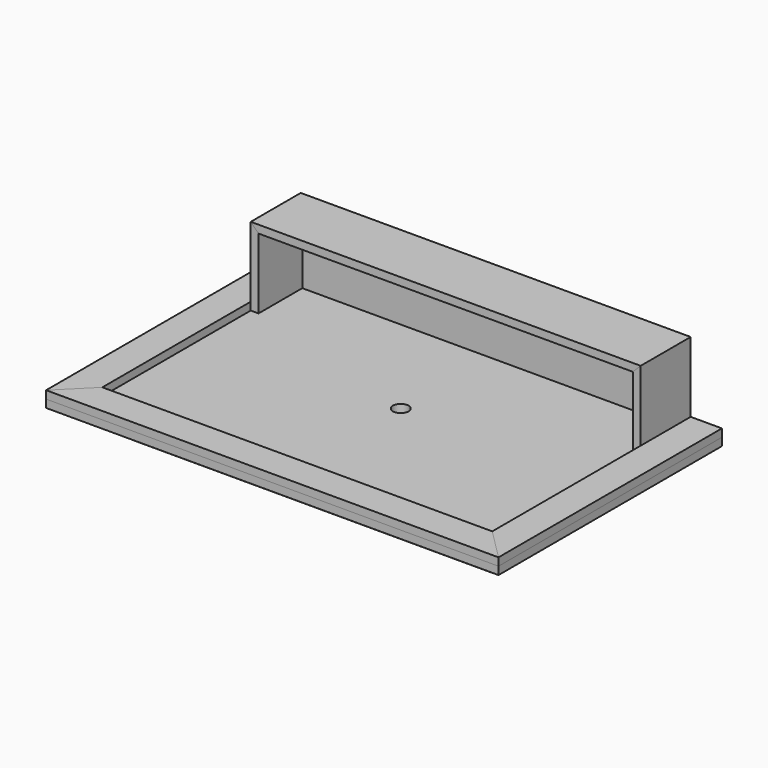
from build123d import *

# Parameters (mm, degrees)
F0_W      = 1470.6092
F0_H      = 907.74012
F1_DEPTH  = 25.4
F2_W      = 1165.8091658585
F2_H      = 720.8011658585
F2_W_2    = 1115.0092
F2_H_2    = 670.0012
F3_DEPTH  = 107.95
F4_R      = 25.4
F5_DEPTH  = 25.4
F6_R      = 9.525
F7_DEPTH  = 720.8011658585
F9_DEPTH  = 25.4
F10_DEPTH = 25.4
F11_DEPTH = 25.4
F12_W     = 1216.6092
F12_H     = 25.4
F13_DEPTH = 254
F14_SIZE  = 25.39999
F16_W     = 1267.4092
F16_H     = 203.2
F17_DEPTH = 25.4
F18_SIZE  = 25.39999


# Not quite as in the source:
# - a fillet or chamfer is up to 0.001 mm smaller than in the source, because OpenCascade refuses the exact size


with BuildPart() as f1:
    # F0 (on Top) → F1 (new body)
    with BuildSketch(Plane.XY):
        with Locations((735.3046, -453.87006)):
            Rectangle(F0_W, F0_H)
    extrude(amount=F1_DEPTH)

    # F2 (on face) → F3 (join)
    with BuildSketch(Plane(origin=(0, 0, 0), x_dir=(1, 0, 0), z_dir=(0, 0, -1))):
        with Locations((735.3046, 385.8005829292)):
            Rectangle(F2_W, F2_H)
        with Locations((735.3046, 385.8005829292)):
            Rectangle(F2_W_2, F2_H_2, mode=Mode.SUBTRACT)
    extrude(amount=F3_DEPTH)

    # F4 (on face) → F5 (cut, through all)
    with BuildSketch(Plane(origin=(0, 0, 0), x_dir=(1, 0, 0), z_dir=(0, 0, -1))):
        with Locations((735.3046, 385.8005829292)):
            Circle(F4_R)
    extrude(amount=-F5_DEPTH, mode=Mode.SUBTRACT)

    # F6 (on face) → F7 (cut, through all)
    with BuildSketch(Plane.XZ.offset(746.2011658585)):
        with Locations((735.3046, -53.975)):
            Circle(F6_R)
        with Locations((241.3000170708, -53.975)):
            Circle(F6_R)
        with Locations((1229.3091829292, -53.975)):
            Circle(F6_R)
    extrude(amount=-F7_DEPTH, mode=Mode.SUBTRACT)


with BuildPart() as f9:
    # F8 (on face) → F9 (new body)
    with BuildSketch(Plane.XY.offset(25.4)):
        Polygon((101.6, 0), (0, 0), (0, -907.74012), (101.6, -806.14012), align=None)
    extrude(amount=F9_DEPTH)


with BuildPart() as f10:
    # F8 (on face) → F10 (new body)
    with BuildSketch(Plane.XY.offset(25.4)):
        Polygon((101.6, -806.14012), (0, -907.74012), (1470.6092, -907.74012), (1369.0092, -806.14012), align=None)
    extrude(amount=F10_DEPTH)


with BuildPart() as f11:
    # F8 (on face) → F11 (new body)
    with BuildSketch(Plane.XY.offset(25.4)):
        Polygon((1369.0092, -806.14012), (1470.6092, -907.74012), (1470.6092, 0), (1369.0092, 0), align=None)
    extrude(amount=F11_DEPTH)


with BuildPart() as f13:
    # F12 (on face) → F13 (new body)
    with BuildSketch(Plane.XY.offset(25.4)):
        Polygon((127, 0), (101.6, 0), (101.6, -203.2), (127, -203.2), (127, -25.4), align=None)
        with Locations((735.3046, -12.7)):
            Rectangle(F12_W, F12_H)
        Polygon((1369.0092, 0), (1343.6092, 0), (1343.6092, -25.4), (1343.6092, -203.2), (1369.0092, -203.2), align=None)
    extrude(amount=F13_DEPTH)

    # F14 (size 25.4 in the source; OpenCascade refuses exactly that, so slightly less here)
    f14_edges = [f13.edges().sort_by_distance(p)[0] for p in [
        (735.3046, -25.4, 279.4),
        (127, -114.3, 279.4),
        (1343.6092, -114.3, 279.4),
    ]]
    chamfer(f14_edges, length=F14_SIZE)


with BuildPart() as f17:
    # F16 (on face) → F17 (new body)
    with BuildSketch(Plane.XY.offset(279.4)):
        with Locations((735.3046, -101.6)):
            Rectangle(F16_W, F16_H)
    extrude(amount=-F17_DEPTH)

    # F18 (size 25.4 in the source; OpenCascade refuses exactly that, so slightly less here)
    f18_edges = [f17.edges().sort_by_distance(p)[0] for p in [
        (101.6, -101.6, 254),
        (735.3046, 0, 254),
        (1369.0092, -101.6, 254),
    ]]
    chamfer(f18_edges, length=F18_SIZE)


solid = Compound([f1.part, f9.part, f10.part, f11.part, f13.part, f17.part])
